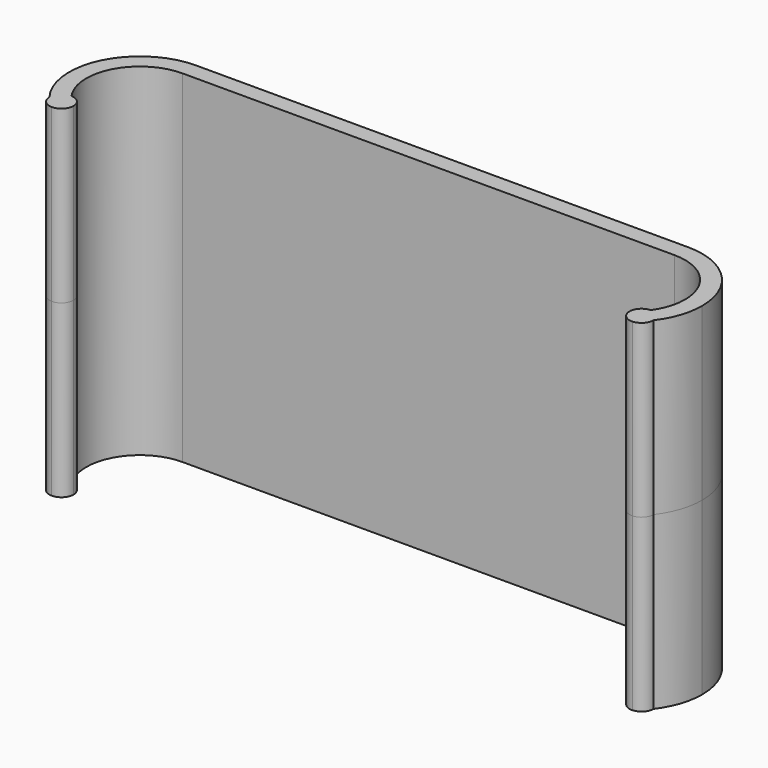
from build123d import *

# Parameters (mm, degrees)
F1_DEPTH = 20


with BuildPart() as f1:
    # F0 (on Top) → F1 (new body, symmetric)
    with BuildSketch(Plane.XY):
        with BuildLine():
            Line((-28.75, 8.25), (-28.75, 6.25))
            Line((-28.75, 6.25), (-23.3648351929, 6.25))
            ThreePointArc((-23.3648351929, 6.25), (-25.8777186767, 7.7338541491), (-28.75, 8.25))
        make_face()
        with BuildLine():
            ThreePointArc((-33.8628873162, -3.5945630182), (-34.2965538339, 2.8806666881), (-28.75, 6.25))
            Line((-28.75, 6.25), (-28.75, 8.25))
            ThreePointArc((-28.75, 8.25), (-36.1429865413, 3.661454629), (-35.3122023742, -5))
            ThreePointArc((-35.3122023742, -5), (-34.8849672334, -3.9905735233), (-33.8628873162, -3.5945630182))
        make_face()
        with BuildLine():
            ThreePointArc((-28.75, 8.25), (-25.8777186767, 7.7338541491), (-23.3648351929, 6.25))
            Line((-23.3648351929, 6.25), (23.3648351929, 6.25))
            ThreePointArc((23.3648351929, 6.25), (25.8777186767, 7.7338541491), (28.75, 8.25))
            Line((28.75, 8.25), (-28.75, 8.25))
        make_face()
        with BuildLine():
            ThreePointArc((-32.5, -5), (-32.8966747104, -4.0211339537), (-33.8628873162, -3.5945630182))
            ThreePointArc((-33.8628873162, -3.5945630182), (-33.2368147022, -4.3509761925), (-32.5, -5))
        make_face()
        with BuildLine():
            ThreePointArc((-32.5, -5), (-33.2368147022, -4.3509761925), (-33.8628873162, -3.5945630182))
            ThreePointArc((-33.8628873162, -3.5945630182), (-34.8849672334, -3.9905735233), (-35.3122023742, -5))
            Line((-35.3122023742, -5), (-32.5, -5))
        make_face()
        with BuildLine():
            ThreePointArc((28.75, 8.25), (25.8777186767, 7.7338541491), (23.3648351929, 6.25))
            Line((23.3648351929, 6.25), (28.75, 6.25))
            Line((28.75, 6.25), (28.75, 8.25))
        make_face()
        with BuildLine():
            ThreePointArc((-33.949315058, -6.4054369818), (-32.9272351408, -6.0094264767), (-32.5, -5))
            Line((-32.5, -5), (-35.3122023742, -5))
            ThreePointArc((-35.3122023742, -5), (-34.672595407, -5.7432885741), (-33.949315058, -6.4054369818))
        make_face()
        with BuildLine():
            ThreePointArc((37, 0), (34.5836309448, 5.8336309448), (28.75, 8.25))
            Line((28.75, 8.25), (28.75, 6.25))
            ThreePointArc((28.75, 6.25), (33.1694173824, 4.4194173824), (35, 0))
            ThreePointArc((35, 0), (34.7089447776, -1.8850668786), (33.8628873162, -3.5945630182))
            ThreePointArc((33.8628873162, -3.5945630182), (34.8849672334, -3.9905735233), (35.3122023742, -5))
            ThreePointArc((35.3122023742, -5), (36.5666703137, -2.6385915194), (37, 0))
        make_face()
        with BuildLine():
            ThreePointArc((-33.949315058, -6.4054369818), (-34.672595407, -5.7432885741), (-35.3122023742, -5))
            ThreePointArc((-35.3122023742, -5), (-34.9155276638, -5.9788660463), (-33.949315058, -6.4054369818))
        make_face()
        with BuildLine():
            ThreePointArc((33.949315058, -6.4054369818), (34.9155276638, -5.9788660463), (35.3122023742, -5))
            ThreePointArc((35.3122023742, -5), (34.672595407, -5.7432885741), (33.949315058, -6.4054369818))
        make_face()
        with BuildLine():
            ThreePointArc((33.949315058, -6.4054369818), (34.672595407, -5.7432885741), (35.3122023742, -5))
            Line((35.3122023742, -5), (32.5, -5))
            ThreePointArc((32.5, -5), (32.9272351408, -6.0094264767), (33.949315058, -6.4054369818))
        make_face()
        with BuildLine():
            Line((32.5, -5), (35.3122023742, -5))
            ThreePointArc((35.3122023742, -5), (34.8849672334, -3.9905735233), (33.8628873162, -3.5945630182))
            ThreePointArc((33.8628873162, -3.5945630182), (33.2368147022, -4.3509761925), (32.5, -5))
        make_face()
        with BuildLine():
            ThreePointArc((33.8628873162, -3.5945630182), (32.8966747104, -4.0211339537), (32.5, -5))
            ThreePointArc((32.5, -5), (33.2368147022, -4.3509761925), (33.8628873162, -3.5945630182))
        make_face()
    extrude(amount=F1_DEPTH, both=True)


solid = f1.part
